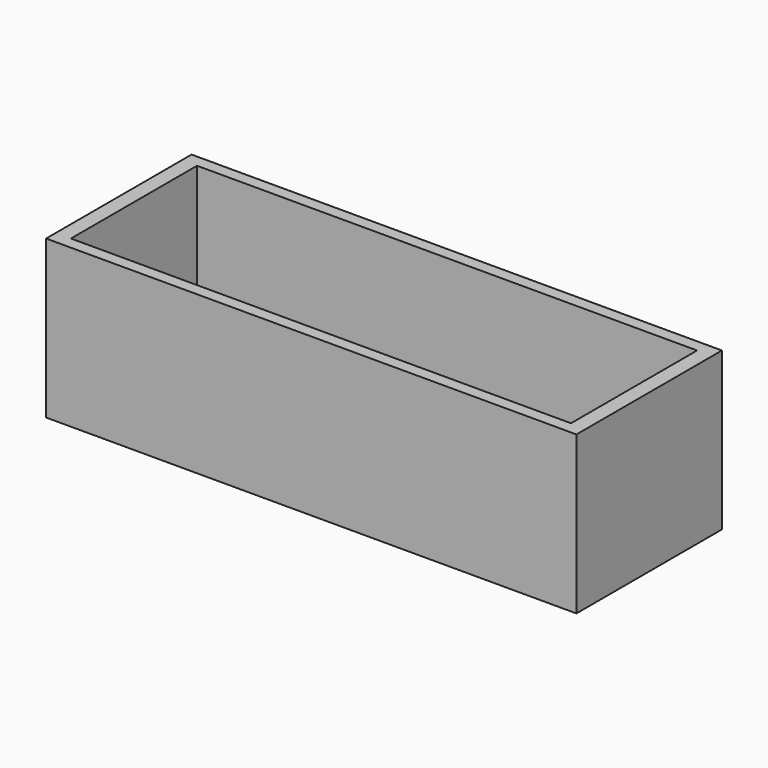
from build123d import *

# Parameters (mm, degrees)
F0_W     = 825
F0_H     = 20
F1_DEPTH = 260
F0_H_2   = 260
F2_DEPTH = 25


# Not quite as in the source:
# - ends of sketch curves that miss each other by under 0.0002 mm in the source are joined
# - a feature names something its author has since deleted; it is built from what else it names


with BuildPart() as f1:
    # F0 (on Top) → F1 (new body)
    with BuildSketch(Plane.XY):
        Polygon((422.5, 130), (422.5, 149.9999940395), (-402.5, 150), (-402.5, 130), align=None)
        Polygon((422.5, -150), (447.5, -150), (447.5, 150), (422.5, 150), (422.5, 130), (422.5, -130), align=None)
        with Locations((10, -140)):
            Rectangle(F0_W, F0_H)
        Polygon((-427.5, -150), (-402.5, -150), (-402.5, -130), (-402.5, 130), (-402.5, 149.9999940395), (-427.5, 150), align=None)
    extrude(amount=F1_DEPTH)

    # F0 (on Top) → F2 (join)
    with BuildSketch(Plane.XY):
        with Locations((10, 0)):
            Rectangle(F0_W, F0_H_2)
    extrude(amount=F2_DEPTH)


solid = f1.part
